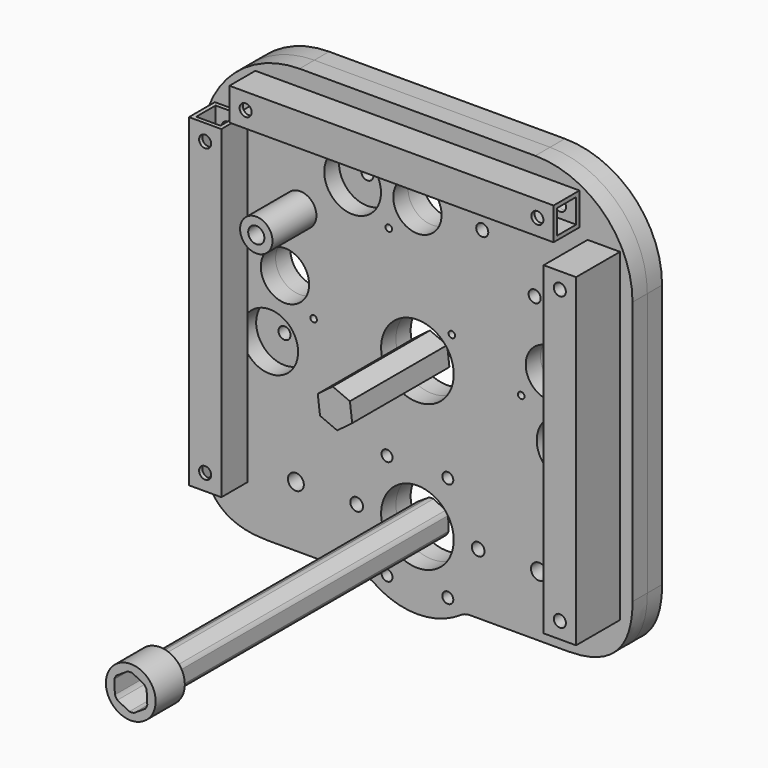
from build123d import *

# Parameters (mm, degrees)
F0_R         = 2.3622
F0_R_2       = 3.1115
F0_R_3       = 2.15265
F0_R_4       = 2.4892
F0_R_5       = 1.27
F0_R_6       = 14.224
F0_R_7       = 9.4615
F1_DEPTH     = 7.239
F2_R         = 6.35
F2_R_2       = 3.175
F3_DEPTH     = 28.7528
F4_W         = 12.7
F4_H         = 127
F4_R         = 2.3622
F5_DEPTH     = 28.7528
F7_DEPTH     = 47.625
F9_DEPTH     = 133.35
F10_T1_DEPTH = 134.239
F11_R        = 6.35
F12_R        = 38.1
F13_R        = 2.3622
F13_R_2      = 3.1115
F13_R_3      = 2.15265
F13_R_4      = 2.4892
F13_R_5      = 11.1125
F13_R_6      = 1.27
F13_R_7      = 14.224
F13_R_8      = 9.4615
F14_DEPTH    = 7.239
F15_W        = 12.7
F15_H        = 127
F15_R        = 2.3622
F16_DEPTH    = 12.7
F17_W        = 127
F17_H        = 12.7
F17_R        = 2.3622
F18_DEPTH    = 12.7
F19_R        = 9.7536
F20_DEPTH    = 14.2875
F21_W        = 9.525
F21_H        = 9.525
F22_DEPTH    = 127
F23_W        = 9.525
F23_H        = 9.525
F24_DEPTH    = 127


# Not quite as in the source:
# - a fillet or chamfer that OpenCascade refuses, or shapes differently, is made with other operations: its cross-section is extruded or revolved along the edge and cut away or added


with BuildPart() as f1:
    # F0 (on Front) → F1 (new body)
    with BuildSketch(Plane.XZ):
        with BuildLine():
            Line((84.2803794373, -81.0133), (84.2803794373, 85.7758))
            Line((84.2803794373, 85.7758), (-84.2803794373, 85.7758))
            Line((-84.2803794373, 85.7758), (-84.2803794373, -81.0133))
            Line((-84.2803794373, -81.0133), (-18.5132722661, -81.0133))
            ThreePointArc((-18.5132722661, -81.0133), (0, -87.3633), (18.5132722661, -81.0133))
            Line((18.5132722661, -81.0133), (84.2803794373, -81.0133))
        make_face()
        with Locations((-73.025, -57.2008)):
            Circle(F0_R, mode=Mode.SUBTRACT)
        with Locations((-47.625, -57.2008)):
            Circle(F0_R_2, mode=Mode.SUBTRACT)
        with Locations((-11.90625, -77.8230299276)):
            Circle(F0_R_3, mode=Mode.SUBTRACT)
        with Locations((-23.8125, -57.2008)):
            Circle(F0_R_4, mode=Mode.SUBTRACT)
        with Locations((-57.8648339281, -12.1407791805)):
            Circle(F0_R, mode=Mode.SUBTRACT)
        with Locations((-11.90625, -36.5785700724)):
            Circle(F0_R_3, mode=Mode.SUBTRACT)
        with Locations((-13.4703841816, -13.4703841816)):
            Circle(F0_R_5, mode=Mode.SUBTRACT)
        with Locations((11.90625, -77.8230299276)):
            Circle(F0_R_3, mode=Mode.SUBTRACT)
        with Locations((0, -57.2008)):
            Circle(F0_R_6, mode=Mode.SUBTRACT)
        with Locations((23.8125, -57.2008)):
            Circle(F0_R_4, mode=Mode.SUBTRACT)
        with Locations((47.625, -57.2008)):
            Circle(F0_R_2, mode=Mode.SUBTRACT)
        with Locations((73.025, -57.2008)):
            Circle(F0_R, mode=Mode.SUBTRACT)
        with Locations((11.90625, -36.5785700724)):
            Circle(F0_R_3, mode=Mode.SUBTRACT)
        with Locations((57.8648339281, -12.1407791805)):
            Circle(F0_R, mode=Mode.SUBTRACT)
        with Locations((-51.8953794373, 12.5477933397)):
            Circle(F0_R_7, mode=Mode.SUBTRACT)
        with Locations((-63.1206995887, 23.773113491)):
            Circle(F0_R_5, mode=Mode.SUBTRACT)
        with Locations((-45.9259249465, 37.2363658598)):
            Circle(F0_R, mode=Mode.SUBTRACT)
        with Locations((-40.670059286, 1.3224731883)):
            Circle(F0_R_5, mode=Mode.SUBTRACT)
        with Locations((-11.2253201513, 42.1654798487)):
            Circle(F0_R_5, mode=Mode.SUBTRACT)
        with Locations((-73.025, 57.0992)):
            Circle(F0_R, mode=Mode.SUBTRACT)
        with Locations((-57.15, 73.0758)):
            Circle(F0_R, mode=Mode.SUBTRACT)
        with Locations((-25.4, 53.3908)):
            Circle(F0_R, mode=Mode.SUBTRACT)
        Circle(F0_R_6, mode=Mode.SUBTRACT)
        with Locations((13.4703841816, 13.4703841816)):
            Circle(F0_R_5, mode=Mode.SUBTRACT)
        with Locations((40.670059286, 1.3224731883)):
            Circle(F0_R_5, mode=Mode.SUBTRACT)
        with Locations((51.8953794373, 12.5477933397)):
            Circle(F0_R_7, mode=Mode.SUBTRACT)
        with Locations((63.1206995887, 23.773113491)):
            Circle(F0_R_5, mode=Mode.SUBTRACT)
        with Locations((45.9259249465, 37.2363658598)):
            Circle(F0_R, mode=Mode.SUBTRACT)
        with Locations((0, 53.3908)):
            Circle(F0_R_7, mode=Mode.SUBTRACT)
        with Locations((25.4, 53.3908)):
            Circle(F0_R, mode=Mode.SUBTRACT)
        with Locations((11.2253201513, 64.6161201513)):
            Circle(F0_R_5, mode=Mode.SUBTRACT)
        with Locations((73.025, 57.0992)):
            Circle(F0_R, mode=Mode.SUBTRACT)
        with Locations((57.15, 73.0758)):
            Circle(F0_R, mode=Mode.SUBTRACT)
    extrude(amount=F1_DEPTH)

    # F10: fillet of radius 25.4 on 2 edges, made by hand

    # F10_s2 → F10_t1 (cut)
    with BuildSketch(Plane.XZ.offset(-63.5)):
        with BuildLine():
            add(Edge.make_bspline(
                [(84.2803794373, -55.6133), (84.2803794373, -81.0133), (58.8803794373, -81.0133)],
                knots=[0, 0, 0, 1, 1, 1], degree=2, weights=[1, 1, 1]))
            Line((58.8803794373, -81.0133), (84.2803794373, -81.0133))
            Line((84.2803794373, -81.0133), (84.2803794373, -55.6133))
        make_face()
        with BuildLine():
            add(Edge.make_bspline(
                [(-84.2803794373, -55.6133), (-84.2803794373, -81.0133), (-58.8803794373, -81.0133)],
                knots=[0, 0, 0, 1, 1, 1], degree=2, weights=[1, 1, 1]))
            Line((-58.8803794373, -81.0133), (-84.2803794373, -81.0133))
            Line((-84.2803794373, -81.0133), (-84.2803794373, -55.6133))
        make_face()
    extrude(amount=F10_T1_DEPTH, mode=Mode.SUBTRACT)

    # F11
    f11_edges = [f1.edges().sort_by_distance(p)[0] for p in [
        (-18.513272, -3.6195, -81.0133),
        (18.513272, -3.6195, -81.0133),
    ]]
    fillet(f11_edges, radius=F11_R)

    # F12
    f12_edges = [f1.edges().sort_by_distance(p)[0] for p in [
        (-84.280379, -3.6195, 85.7758),
        (84.280379, -3.6195, 85.7758),
    ]]
    fillet(f12_edges, radius=F12_R)


with BuildPart() as f3:
    # F2 (on face) → F3 (new body)
    with BuildSketch(Plane.XZ.offset(7.239)):
        with Locations((-45.9259249465, 37.2363658598)):
            Circle(F2_R)
        with Locations((-45.9259249465, 37.2363658598)):
            Circle(F2_R_2, mode=Mode.SUBTRACT)
    extrude(amount=F3_DEPTH)


with BuildPart() as f5:
    # F4 (on face) → F5 (new body, through all)
    with BuildSketch(Plane.XZ.offset(7.239)):
        with Locations((73.025, -0.0508)):
            Rectangle(F4_W, F4_H)
        with Locations((73.025, -57.2008)):
            Circle(F4_R, mode=Mode.SUBTRACT)
        with Locations((73.025, 57.0992)):
            Circle(F4_R, mode=Mode.SUBTRACT)
    extrude(amount=F5_DEPTH)


with BuildPart() as f7:
    # F6 (on face) → F7 (new body)
    with BuildSketch(Plane.XZ.offset(7.239)):
        Polygon((0.8878003498, -7.2784025632), (6.7471816936, -2.8703436252), (5.8593813438, 4.408058938), (-0.8878003498, 7.2784025632), (-6.7471816936, 2.8703436252), (-5.8593813438, -4.408058938), align=None)
    extrude(amount=F7_DEPTH)


with BuildPart() as f9:
    # F8 (on face) → F9 (new body)
    with BuildSketch(Plane.XZ.offset(7.239)):
        with BuildLine():
            Line((1.2297627695, -63.9649191984), (5.6574931463, -61.1069997261))
            ThreePointArc((5.6574931463, -61.1069997261), (6.1169625258, -60.3390151707), (6.4727804448, -59.5178538002))
            Line((6.4727804448, -59.5178538002), (6.2116147682, -54.2543670766))
            ThreePointArc((6.2116147682, -54.2543670766), (5.7762553233, -53.472462644), (5.2430176753, -52.7537346018))
            Line((5.2430176753, -52.7537346018), (0.5541216219, -50.3481673506))
            ThreePointArc((0.5541216219, -50.3481673506), (-0.3407072025, -50.3342474733), (-1.2297627695, -50.4366808016))
            Line((-1.2297627695, -50.4366808016), (-5.6574931463, -53.2946002739))
            ThreePointArc((-5.6574931463, -53.2946002739), (-6.1169625258, -54.0625848293), (-6.4727804448, -54.8837461998))
            Line((-6.4727804448, -54.8837461998), (-6.2116147682, -60.1472329234))
            ThreePointArc((-6.2116147682, -60.1472329234), (-5.7762553233, -60.929137356), (-5.2430176753, -61.6478653982))
            Line((-5.2430176753, -61.6478653982), (-0.5541216219, -64.0534326494))
            ThreePointArc((-0.5541216219, -64.0534326494), (0.3407072025, -64.0673525267), (1.2297627695, -63.9649191984))
        make_face()
    extrude(amount=F9_DEPTH)


with BuildPart() as f14:
    # F13 (on face) → F14 (new body)
    with BuildSketch(Plane.XZ.offset(7.239)):
        with BuildLine():
            add(Edge.make_bspline(
                [(58.8803794373, -81.0133), (60.3638077373, -81.0133), (61.846545506, -80.9627619053), (63.3276626583, -80.8555743869), (64.8040734271, -80.6842485298), (66.2705596958, -80.4400438138), (67.719781852, -80.113053691), (69.6606517662, -79.5398434055), (70.175270504, -79.3744504286), (70.6857251043, -79.1962557829), (71.1914268059, -79.0048026522), (71.6917208065, -78.7996641317), (72.185894623, -78.580464911), (72.9435661798, -78.2173205554), (73.2118244175, -78.0833122708), (73.4778326847, -77.9448351063), (73.7414558157, -77.801846904), (74.0025554116, -77.6543145731), (74.2609907071, -77.5022156734), (75.0466303898, -77.0206945775), (75.564621459, -76.6761468216), (76.0692584522, -76.3118388215), (76.559270294, -75.9279041794), (77.0334770511, -75.5247037665), (77.4908179571, -75.1028614802), (78.5819199856, -74.0117594517), (79.1946118608, -73.3210751105), (79.7652831629, -72.5943518866), (80.2923948477, -71.8353279793), (80.7756690879, -71.0481164752), (81.2157631862, -70.236975882), (81.8475443483, -68.9188151857), (82.066743569, -68.4246413692), (82.2718820895, -67.9243473686), (82.4633352202, -67.418645667), (82.6415298659, -66.9081910667), (82.8069228428, -66.3935723289), (83.3801331283, -64.4527024147), (83.7071232511, -63.0034802585), (83.9513279671, -61.5369939898), (84.1226538242, -60.060583221), (84.2298413426, -58.5794660687), (84.2803794373, -57.0967283), (84.2803794373, -55.6133)],
                knots=[0, 0, 0, 0, 0, 0, 0, 0, 0.2518137599, 0.2518137599, 0.2518137599, 0.2518137599, 0.2518137599, 0.2518137599, 0.3435515123, 0.3435515123, 0.3435515123, 0.3435515123, 0.3435515123, 0.3435515123, 0.39445255, 0.39445255, 0.39445255, 0.39445255, 0.39445255, 0.39445255, 0.4999888387, 0.4999888387, 0.4999888387, 0.4999888387, 0.4999888387, 0.4999888387, 0.6564201333, 0.6564201333, 0.6564201333, 0.6564201333, 0.6564201333, 0.6564201333, 0.7481654571, 0.7481654571, 0.7481654571, 0.7481654571, 0.7481654571, 0.7481654571, 1, 1, 1, 1, 1, 1, 1, 1], degree=7))
            Line((84.2803794373, -55.6133), (84.2803794373, 47.6758))
            ThreePointArc((84.2803794373, 47.6758), (73.1211478005, 74.6165683632), (46.1803794373, 85.7758))
            Line((46.1803794373, 85.7758), (-46.1803794373, 85.7758))
            ThreePointArc((-46.1803794373, 85.7758), (-73.1211478005, 74.6165683632), (-84.2803794373, 47.6758))
            Line((-84.2803794373, 47.6758), (-84.2803794373, -55.6133))
            add(Edge.make_bspline(
                [(-58.8803794373, -81.0133), (-60.3638077373, -81.0133), (-61.846545506, -80.9627619053), (-63.3276626583, -80.8555743869), (-64.8040734271, -80.6842485298), (-66.2705596958, -80.4400438138), (-67.719781852, -80.113053691), (-69.6606517662, -79.5398434055), (-70.175270504, -79.3744504286), (-70.6857251043, -79.1962557829), (-71.1914268059, -79.0048026522), (-71.6917208065, -78.7996641317), (-72.185894623, -78.580464911), (-72.9435661798, -78.2173205554), (-73.2118244175, -78.0833122708), (-73.4778326847, -77.9448351063), (-73.7414558157, -77.801846904), (-74.0025554116, -77.6543145731), (-74.2609907071, -77.5022156734), (-75.0466303898, -77.0206945775), (-75.564621459, -76.6761468216), (-76.0692584522, -76.3118388215), (-76.559270294, -75.9279041794), (-77.0334770511, -75.5247037665), (-77.4908179571, -75.1028614802), (-78.5819199856, -74.0117594517), (-79.1946118609, -73.3210751105), (-79.7652831629, -72.5943518866), (-80.2923948477, -71.8353279793), (-80.7756690879, -71.0481164752), (-81.2157631862, -70.236975882), (-81.8475443483, -68.9188151857), (-82.066743569, -68.4246413692), (-82.2718820895, -67.9243473686), (-82.4633352202, -67.418645667), (-82.6415298659, -66.9081910667), (-82.8069228428, -66.3935723289), (-83.3801331283, -64.4527024147), (-83.7071232511, -63.0034802585), (-83.9513279671, -61.5369939898), (-84.1226538242, -60.060583221), (-84.2298413426, -58.5794660687), (-84.2803794373, -57.0967283), (-84.2803794373, -55.6133)],
                knots=[0, 0, 0, 0, 0, 0, 0, 0, 0.2518137599, 0.2518137599, 0.2518137599, 0.2518137599, 0.2518137599, 0.2518137599, 0.3435515123, 0.3435515123, 0.3435515123, 0.3435515123, 0.3435515123, 0.3435515123, 0.39445255, 0.39445255, 0.39445255, 0.39445255, 0.39445255, 0.39445255, 0.4999888387, 0.4999888387, 0.4999888387, 0.4999888387, 0.4999888387, 0.4999888387, 0.6564201333, 0.6564201333, 0.6564201333, 0.6564201333, 0.6564201333, 0.6564201333, 0.7481654571, 0.7481654571, 0.7481654571, 0.7481654571, 0.7481654571, 0.7481654571, 1, 1, 1, 1, 1, 1, 1, 1], degree=7))
            Line((-58.8803794373, -81.0133), (-20.5763517174, -81.0133))
            ThreePointArc((-20.5763517174, -81.0133), (-18.7038388743, -81.2956649045), (-16.9978557666, -82.1176478261))
            ThreePointArc((-16.9978557666, -82.1176478261), (0, -87.3633), (16.9978557666, -82.1176478261))
            ThreePointArc((16.9978557666, -82.1176478261), (18.7038388743, -81.2956649045), (20.5763517174, -81.0133))
            Line((20.5763517174, -81.0133), (58.8803794373, -81.0133))
        make_face()
        with Locations((-73.025, -57.2008)):
            Circle(F13_R, mode=Mode.SUBTRACT)
        with Locations((-47.625, -57.2008)):
            Circle(F13_R_2, mode=Mode.SUBTRACT)
        with Locations((-11.90625, -77.8230299276)):
            Circle(F13_R_3, mode=Mode.SUBTRACT)
        with Locations((-23.8125, -57.2008)):
            Circle(F13_R_4, mode=Mode.SUBTRACT)
        with Locations((-57.8648339281, -12.1407791805)):
            Circle(F13_R_5, mode=Mode.SUBTRACT)
        with Locations((-11.90625, -36.5785700724)):
            Circle(F13_R_3, mode=Mode.SUBTRACT)
        with Locations((-13.4703841816, -13.4703841816)):
            Circle(F13_R_6, mode=Mode.SUBTRACT)
        with Locations((11.90625, -77.8230299276)):
            Circle(F13_R_3, mode=Mode.SUBTRACT)
        with Locations((0, -57.2008)):
            Circle(F13_R_7, mode=Mode.SUBTRACT)
        with Locations((23.8125, -57.2008)):
            Circle(F13_R_4, mode=Mode.SUBTRACT)
        with Locations((47.625, -57.2008)):
            Circle(F13_R_2, mode=Mode.SUBTRACT)
        with Locations((73.025, -57.2008)):
            Circle(F13_R, mode=Mode.SUBTRACT)
        with Locations((11.90625, -36.5785700724)):
            Circle(F13_R_3, mode=Mode.SUBTRACT)
        with Locations((57.8648339281, -12.1407791805)):
            Circle(F13_R_5, mode=Mode.SUBTRACT)
        with Locations((-51.8953794373, 12.5477933397)):
            Circle(F13_R_8, mode=Mode.SUBTRACT)
        with Locations((-63.1206995887, 23.773113491)):
            Circle(F13_R_6, mode=Mode.SUBTRACT)
        with Locations((-45.9259249465, 37.2363658598)):
            Circle(F13_R, mode=Mode.SUBTRACT)
        with Locations((-40.670059286, 1.3224731883)):
            Circle(F13_R_6, mode=Mode.SUBTRACT)
        with Locations((-11.2253201513, 42.1654798487)):
            Circle(F13_R_6, mode=Mode.SUBTRACT)
        with Locations((-73.025, 57.0992)):
            Circle(F13_R, mode=Mode.SUBTRACT)
        with Locations((-57.15, 73.0758)):
            Circle(F13_R, mode=Mode.SUBTRACT)
        with Locations((-25.4, 53.3908)):
            Circle(F13_R_5, mode=Mode.SUBTRACT)
        Circle(F13_R_7, mode=Mode.SUBTRACT)
        with Locations((13.4703841816, 13.4703841816)):
            Circle(F13_R_6, mode=Mode.SUBTRACT)
        with Locations((40.670059286, 1.3224731883)):
            Circle(F13_R_6, mode=Mode.SUBTRACT)
        with Locations((51.8953794373, 12.5477933397)):
            Circle(F13_R_8, mode=Mode.SUBTRACT)
        with Locations((63.1206995887, 23.773113491)):
            Circle(F13_R_6, mode=Mode.SUBTRACT)
        with Locations((45.9259249465, 37.2363658598)):
            Circle(F13_R, mode=Mode.SUBTRACT)
        with Locations((0, 53.3908)):
            Circle(F13_R_8, mode=Mode.SUBTRACT)
        with Locations((25.4, 53.3908)):
            Circle(F13_R, mode=Mode.SUBTRACT)
        with Locations((11.2253201513, 64.6161201513)):
            Circle(F13_R_6, mode=Mode.SUBTRACT)
        with Locations((73.025, 57.0992)):
            Circle(F13_R, mode=Mode.SUBTRACT)
        with Locations((57.15, 73.0758)):
            Circle(F13_R, mode=Mode.SUBTRACT)
    extrude(amount=F14_DEPTH)


with BuildPart() as f16:
    # F15 (on face) → F16 (new body)
    with BuildSketch(Plane.XZ.offset(14.478)):
        with Locations((-73.025, -0.0508)):
            Rectangle(F15_W, F15_H)
        with Locations((-73.025, -57.2008)):
            Circle(F15_R, mode=Mode.SUBTRACT)
        with Locations((-73.025, 57.0992)):
            Circle(F15_R, mode=Mode.SUBTRACT)
    extrude(amount=F16_DEPTH)

    # F21 (on face) → F22 (cut, through all)
    with BuildSketch(Plane.XY.offset(63.4492)):
        with Locations((-73.025, -20.828)):
            Rectangle(F21_W, F21_H)
    extrude(amount=-F22_DEPTH, mode=Mode.SUBTRACT)


with BuildPart() as f18:
    # F17 (on face) → F18 (new body)
    with BuildSketch(Plane.XZ.offset(14.478)):
        with Locations((0, 73.0758)):
            Rectangle(F17_W, F17_H)
        with Locations((-57.15, 73.0758)):
            Circle(F17_R, mode=Mode.SUBTRACT)
        with Locations((57.15, 73.0758)):
            Circle(F17_R, mode=Mode.SUBTRACT)
    extrude(amount=F18_DEPTH)

    # F23 (on face) → F24 (cut, through all)
    with BuildSketch(Plane(origin=(-63.5, 0, 0), x_dir=(0, -1, 0), z_dir=(-1, 0, 0))):
        with Locations((20.828, 73.0758)):
            Rectangle(F23_W, F23_H)
    extrude(amount=-F24_DEPTH, mode=Mode.SUBTRACT)


with BuildPart() as f20:
    # F19 (on face) → F20 (new body)
    with BuildSketch(Plane.XZ.offset(140.589)):
        with Locations((0, -57.2008)):
            Circle(F19_R)
        with BuildLine():
            ThreePointArc((-5.2430176753, -61.6478653982), (-5.7762553233, -60.929137356), (-6.2116147682, -60.1472329234))
            Line((-6.2116147682, -60.1472329234), (-6.4727804448, -54.8837461998))
            ThreePointArc((-6.4727804448, -54.8837461998), (-6.1169625258, -54.0625848293), (-5.6574931463, -53.2946002739))
            Line((-5.6574931463, -53.2946002739), (-1.2297627695, -50.4366808016))
            ThreePointArc((-1.2297627695, -50.4366808016), (-0.3407072025, -50.3342474733), (0.5541216219, -50.3481673506))
            Line((0.5541216219, -50.3481673506), (5.2430176753, -52.7537346018))
            ThreePointArc((5.2430176753, -52.7537346018), (5.7762553233, -53.472462644), (6.2116147682, -54.2543670766))
            Line((6.2116147682, -54.2543670766), (6.4727804448, -59.5178538002))
            ThreePointArc((6.4727804448, -59.5178538002), (6.1169625258, -60.3390151707), (5.6574931463, -61.1069997261))
            Line((5.6574931463, -61.1069997261), (1.2297627695, -63.9649191984))
            ThreePointArc((1.2297627695, -63.9649191984), (0.3407072025, -64.0673525267), (-0.5541216219, -64.0534326494))
            Line((-0.5541216219, -64.0534326494), (-5.2430176753, -61.6478653982))
        make_face(mode=Mode.SUBTRACT)
    extrude(amount=F20_DEPTH)


solid = Compound([f1.part, f3.part, f5.part, f7.part, f9.part, f14.part, f16.part, f18.part, f20.part])
